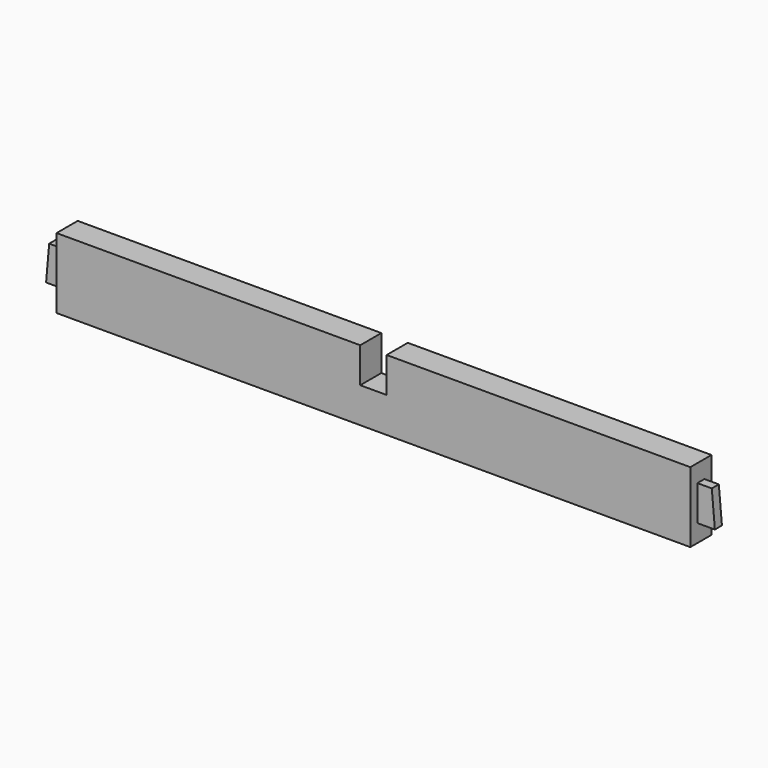
from build123d import *

# Parameters (mm, degrees)
F0_W        = 457.2
F0_H        = 50.8
F1_DEPTH    = 9.525
F2_W        = 19.05
F2_H        = 19.05
F3_DEPTH    = 25.4
F4_W        = 6.35
F4_H        = 25.4
F5_DEPTH    = 12.7
F6_W        = 6.35
F6_H        = 25.4
F7_DEPTH    = 12.7
F8_T1_DEPTH = 142.2021954046


# Not quite as in the source:
# - a fillet or chamfer that OpenCascade refuses, or shapes differently, is made with other operations: its cross-section is extruded or revolved along the edge and cut away or added
# - a feature names something its author has since deleted; it is built from what else it names


with BuildPart() as f1:
    # F0 (on Front) → F1 (new body, symmetric)
    with BuildSketch(Plane.XZ):
        Rectangle(F0_W, F0_H)
    extrude(amount=F1_DEPTH, both=True)

    # F2 (on face) → F3 (cut, symmetric)
    with BuildSketch(Plane.XY.offset(25.4)):
        Rectangle(F2_W, F2_H)
    extrude(amount=F3_DEPTH, both=True, mode=Mode.SUBTRACT)

    # F4 (on face) → F5 (join, symmetric)
    with BuildSketch(Plane.YZ.offset(228.6)):
        Rectangle(F4_W, F4_H)
    extrude(amount=F5_DEPTH, both=True)

    # F6 (on face) → F7 (join, symmetric)
    with BuildSketch(Plane(origin=(-228.6, 0, 0), x_dir=(0, -1, 0), z_dir=(-1, 0, 0))):
        Rectangle(F6_W, F6_H)
    extrude(amount=F7_DEPTH, both=True)

    # F8: chamfer of 2.286 x 26.1290995641 on 2 edges, made by hand

    # F8_s2 → F8_t1 (cut)
    with BuildSketch(Plane.XZ.offset(-71.1010977023)):
        Polygon((-239.014, 12.7), (-241.3, -13.4290995641), (-241.3, 12.7), align=None)
        Polygon((239.014, 12.7), (241.3, -13.4290995641), (241.3, 12.7), align=None)
    extrude(amount=F8_T1_DEPTH, mode=Mode.SUBTRACT)


solid = f1.part
